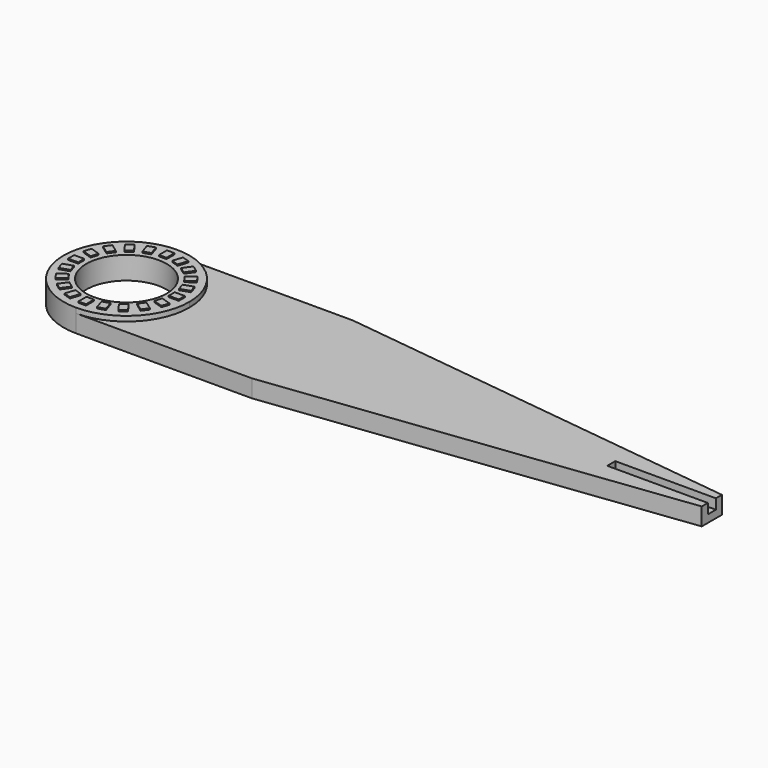
from build123d import *

# Parameters (mm, degrees)
F0_R         = 8
F1_DEPTH     = 3.5
F2_R         = 8
F3_DEPTH     = 1
F4_W         = 1.5
F4_H         = 2
F4_W_2       = 2
F4_H_2       = 1.5
F5_DEPTH     = 0.25
F6_W         = 20
F6_H         = 2
F7_DEPTH     = 2
F8_TEXT_SIZE = 20.8426581122
F9_DEPTH     = 1


# Not quite as in the source:
# - Text() gives the source's letters only with a copy of the font that has no kerning and outlines rounded to 1/6400 em; it was checked with that copy


with BuildPart() as f1:
    # F0 (on Top) → F1 (new body)
    with BuildSketch(Plane.XY):
        with BuildLine():
            ThreePointArc((0, -12.5), (8.8388347648, -8.8388347648), (12.5, 0))
            ThreePointArc((12.5, 0), (8.8388347648, 8.8388347648), (0, 12.5))
            ThreePointArc((0, 12.5), (-12.5, 0), (0, -12.5))
        make_face()
        Circle(F0_R, mode=Mode.SUBTRACT)
        with BuildLine():
            ThreePointArc((0, 12.5), (8.8388347648, 8.8388347648), (12.5, 0))
            ThreePointArc((12.5, 0), (8.8388347648, -8.8388347648), (0, -12.5))
            Line((0, -12.5), (35, -12.5))
            Line((35, -12.5), (116.3887844346, -2.5067138408))
            Line((116.3887844346, -2.5067138408), (116.3887844346, 2.5067138408))
            Line((116.3887844346, 2.5067138408), (35, 12.5))
            Line((35, 12.5), (0, 12.5))
        make_face()
    extrude(amount=F1_DEPTH)

    # F2 (on face) → F3 (join)
    with BuildSketch(Plane.XY.offset(3.5)):
        with BuildLine():
            ThreePointArc((0, -12.5), (8.8388347648, -8.8388347648), (12.5, 0))
            ThreePointArc((12.5, 0), (8.8388347648, 8.8388347648), (0, 12.5))
            ThreePointArc((0, 12.5), (-12.5, 0), (0, -12.5))
        make_face()
        Circle(F2_R, mode=Mode.SUBTRACT)
    extrude(amount=F3_DEPTH)

    # F4 (on face) → F5 (join)
    with BuildSketch(Plane.XY.offset(4.5)):
        with Locations((0, 10)):
            Rectangle(F4_W, F4_H)
        Polygon((-2.6858945509, 10.693384425), (-4.1124793253, 10.2298589335), (-3.4944453366, 8.3277459009), (-2.0678605622, 8.7912713924), align=None)
        Polygon((-5.8588750294, 9.3400258773), (-7.072400521, 8.4583479989), (-5.8968300164, 6.8403140102), (-4.6833045249, 7.7219918886), align=None)
        Polygon((-8.4583479989, 7.072400521), (-9.3400258773, 5.8588750294), (-7.7219918886, 4.6833045249), (-6.8403140102, 5.8968300164), align=None)
        with Locations((-10, 0)):
            Rectangle(F4_W_2, F4_H_2)
        Polygon((-10.693384425, -2.6858945509), (-10.2298589335, -4.1124793253), (-8.3277459009, -3.4944453366), (-8.7912713924, -2.0678605622), align=None)
        Polygon((-9.3400258773, -5.8588750294), (-8.4583479989, -7.072400521), (-6.8403140102, -5.8968300164), (-7.7219918886, -4.6833045249), align=None)
        Polygon((-7.072400521, -8.4583479989), (-5.8588750294, -9.3400258773), (-4.6833045249, -7.7219918886), (-5.8968300164, -6.8403140102), align=None)
        Polygon((-4.1124793253, -10.2298589335), (-2.6858945509, -10.693384425), (-2.0678605622, -8.7912713924), (-3.4944453366, -8.3277459009), align=None)
        with Locations((0, -10)):
            Rectangle(F4_W, F4_H)
        Polygon((2.6858945509, -10.693384425), (4.1124793253, -10.2298589335), (3.4944453366, -8.3277459009), (2.0678605622, -8.7912713924), align=None)
        Polygon((5.8588750294, -9.3400258773), (7.072400521, -8.4583479989), (5.8968300164, -6.8403140102), (4.6833045249, -7.7219918886), align=None)
        Polygon((8.4583479989, -7.072400521), (9.3400258773, -5.8588750294), (7.7219918886, -4.6833045249), (6.8403140102, -5.8968300164), align=None)
        Polygon((10.2298589335, -4.1124793253), (10.693384425, -2.6858945509), (8.7912713924, -2.0678605622), (8.3277459009, -3.4944453366), align=None)
        with Locations((10, 0)):
            Rectangle(F4_W_2, F4_H_2)
        Polygon((10.693384425, 2.6858945509), (10.2298589335, 4.1124793253), (8.3277459009, 3.4944453366), (8.7912713924, 2.0678605622), align=None)
        Polygon((9.3400258773, 5.8588750294), (8.4583479989, 7.072400521), (6.8403140102, 5.8968300164), (7.7219918886, 4.6833045249), align=None)
        Polygon((7.072400521, 8.4583479989), (5.8588750294, 9.3400258773), (4.6833045249, 7.7219918886), (5.8968300164, 6.8403140102), align=None)
        Polygon((4.1124793253, 10.2298589335), (2.6858945509, 10.693384425), (2.0678605622, 8.7912713924), (3.4944453366, 8.3277459009), align=None)
        Polygon((-10.2298589335, 4.1124793253), (-10.693384425, 2.6858945509), (-8.7912713924, 2.0678605622), (-8.3277459009, 3.4944453366), align=None)
    extrude(amount=F5_DEPTH)

    # F6 (on face) → F7 (cut)
    with BuildSketch(Plane.XY.offset(3.5)):
        with Locations((106.3887844346, 0.0067138408)):
            Rectangle(F6_W, F6_H)
    extrude(amount=-F7_DEPTH, mode=Mode.SUBTRACT)

    # F8 (on face) → F9 (cut)
    with BuildSketch(Plane(origin=(0, 0, 0), x_dir=(1, 0, 0), z_dir=(0, 0, -1))):
        with Locations((14.1043374958, -7.5033569204)):
            Text('Esther', F8_TEXT_SIZE, font='Open Sans', text_align=(TextAlign.LEFT, TextAlign.BOTTOM))
    extrude(amount=-F9_DEPTH, mode=Mode.SUBTRACT)


solid = f1.part
